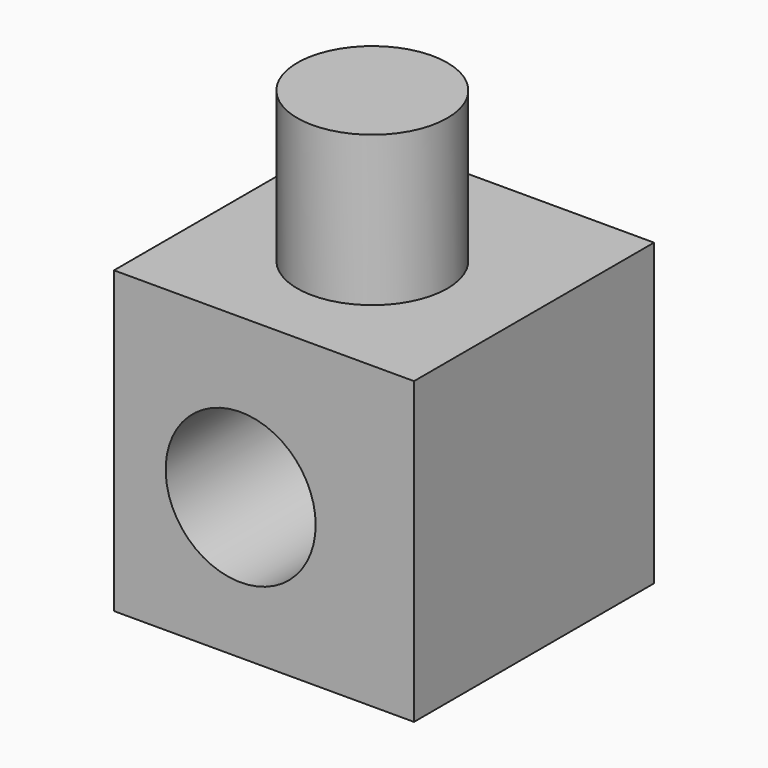
from build123d import *

# Parameters (mm, degrees)
F0_W     = 100
F0_H     = 100
F1_DEPTH = 100
F4_R     = 25
F5_DEPTH = 50
F8_D     = 50


# Not quite as in the source:
# - the program builds the solid bodies; features that only make, move or delete a surface that nothing else refers to are left out


with BuildPart() as f1:
    # F0 (on Front) → F1 (new body)
    with BuildSketch(Plane.XZ):
        with Locations((50, 50)):
            Rectangle(F0_W, F0_H)
    extrude(amount=F1_DEPTH)

    # F4 (on face) → F5 (join)
    with BuildSketch(Plane.XY.offset(100)):
        with Locations((49.1654276848, -53.809389472)):
            Circle(F4_R)
    extrude(amount=F5_DEPTH)

    # F8 (through all)
    with Locations(Plane(origin=(0, 0, 0), x_dir=(-1, 0, 0), z_dir=(0, 1, 0))):
        with Locations((-42.2243028879, 47.1359044313)):
            Hole(F8_D / 2)


solid = f1.part
